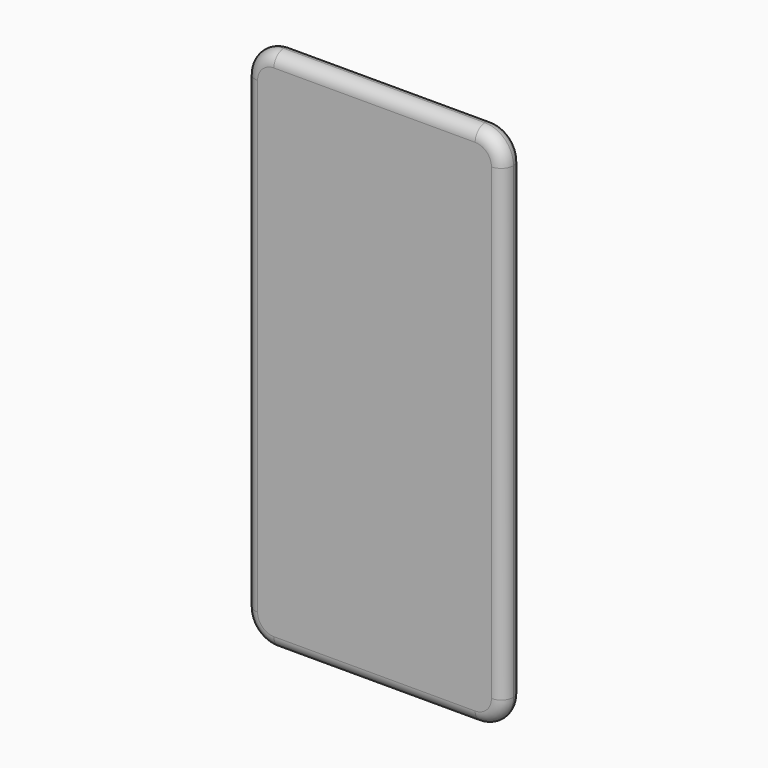
from build123d import *

# Parameters (mm, degrees)
F0_W         = 77.724
F0_H         = 157.988
F1_DEPTH     = 7.112
F2_R         = 8.5849434278
F3_R         = 3.6792614691
F4_T1_DEPTH  = 60.5541131444
F4_T3_DEPTH  = 140.8181131444
F4_T6_ANGLE  = 90
F4_T8_ANGLE  = 90
F4_T10_ANGLE = 90
F4_T12_ANGLE = 90


# Not quite as in the source:
# - a fillet or chamfer that OpenCascade refuses, or shapes differently, is made with other operations: its cross-section is extruded or revolved along the edge and cut away or added


with BuildPart() as f1:
    # F0 (on Front) → F1 (new body)
    with BuildSketch(Plane.XZ):
        with Locations((-9.6872102137, -28.5588150506)):
            Rectangle(F0_W, F0_H)
    extrude(amount=F1_DEPTH)

    # F2
    f2_edges = [f1.edges().sort_by_distance(p)[0] for p in [
        (-48.54921, -3.556, 50.435185),
        (-48.54921, -3.556, -107.552815),
        (29.17479, -3.556, -107.552815),
        (29.17479, -3.556, 50.435185),
    ]]
    fillet(f2_edges, radius=F2_R)

    # F3
    f3_edges = [f1.edges().sort_by_distance(p)[0] for p in [
        (-9.68721, -7.112, 50.435185),
    ]]
    fillet(f3_edges, radius=F3_R)

    # F4: fillet of radius 3.6792614691 on 1 edges, made by hand

    # F4_s2 → F4_t1 (cut)
    with BuildSketch(Plane.YZ.offset(-39.9642667859)):
        with BuildLine():
            ThreePointArc((0, 46.7641917052), (-0.9918847458, 49.2771523705), (-3.4327385309, 50.4351849494))
            Line((-3.4327385309, 50.4351849494), (-3.4278080722, 50.5086048143))
            ThreePointArc((-3.4278080722, 50.5086048143), (-1.7163692655, 50.5087701788), (0, 50.5087701788))
            Line((0, 50.5087701788), (0.0735852294, 50.4351849494))
            Line((0.0735852294, 50.4351849494), (0.0735852294, 46.7641917052))
            Line((0.0735852294, 46.7641917052), (0, 46.7641917052))
        make_face()
        with BuildLine():
            ThreePointArc((-3.4327385309, -107.5528150506), (-0.9918847458, -106.3947824717), (0, -103.8818218065))
            Line((0, -103.8818218065), (0.0735852294, -103.8818218065))
            Line((0.0735852294, -103.8818218065), (0.0735852294, -107.5528150506))
            Line((0.0735852294, -107.5528150506), (0, -107.62640028))
            ThreePointArc((0, -107.62640028), (-1.7163692655, -107.62640028), (-3.4278080722, -107.6262349155))
            Line((-3.4278080722, -107.6262349155), (-3.4327385309, -107.5528150506))
        make_face()
    extrude(amount=F4_T1_DEPTH, mode=Mode.SUBTRACT)

    # F4_s4 → F4_t3 (cut)
    with BuildSketch(Plane.XY.offset(-98.9678716228)):
        with BuildLine():
            ThreePointArc((-44.8782169695, 0), (-47.3911776348, -0.9918847458), (-48.5492102137, -3.4327385309))
            Line((-48.5492102137, -3.4327385309), (-48.6226300785, -3.4278080722))
            ThreePointArc((-48.6226300785, -3.4278080722), (-48.622795443, -1.7163692655), (-48.622795443, 0))
            Line((-48.622795443, 0), (-48.5492102137, 0.0735852294))
            Line((-48.5492102137, 0.0735852294), (-44.8782169695, 0.0735852294))
            Line((-44.8782169695, 0.0735852294), (-44.8782169695, 0))
        make_face()
        with BuildLine():
            ThreePointArc((25.5037965422, 0), (28.0167572074, -0.9918847458), (29.1747897863, -3.4327385309))
            Line((29.1747897863, -3.4327385309), (29.2482096512, -3.4278080722))
            ThreePointArc((29.2482096512, -3.4278080722), (29.2483750157, -1.7163692655), (29.2483750157, 0))
            Line((29.2483750157, 0), (29.1747897863, 0.0735852294))
            Line((29.1747897863, 0.0735852294), (25.5037965422, 0.0735852294))
            Line((25.5037965422, 0.0735852294), (25.5037965422, 0))
        make_face()
    extrude(amount=F4_T3_DEPTH, mode=Mode.SUBTRACT)

    # F4_s5 → F4_t6 (revolve, cut)
    with BuildSketch(Plane.XY.offset(41.8502415216)):
        with BuildLine():
            ThreePointArc((25.5037965422, 0), (28.0167572074, -0.9918847458), (29.1747897863, -3.4327385309))
            Line((29.1747897863, -3.4327385309), (29.2482096512, -3.4278080722))
            ThreePointArc((29.2482096512, -3.4278080722), (29.2483750157, -1.7163692655), (29.2483750157, 0))
            Line((29.2483750157, 0), (29.1747897863, 0.0735852294))
            Line((29.1747897863, 0.0735852294), (25.5037965422, 0.0735852294))
            Line((25.5037965422, 0.0735852294), (25.5037965422, 0))
        make_face()
    revolve(axis=Axis((20.5898463585, 0, 41.8502415216), (0, -1, 0)), revolution_arc=F4_T6_ANGLE, mode=Mode.SUBTRACT)

    # F4_s7 → F4_t8 (revolve, cut)
    with BuildSketch(Plane.YZ.offset(-39.9642667859)):
        with BuildLine():
            ThreePointArc((0, 46.7641917052), (-0.9918847458, 49.2771523705), (-3.4327385309, 50.4351849494))
            Line((-3.4327385309, 50.4351849494), (-3.4278080722, 50.5086048143))
            ThreePointArc((-3.4278080722, 50.5086048143), (-1.7163692655, 50.5087701788), (0, 50.5087701788))
            Line((0, 50.5087701788), (0.0735852294, 50.4351849494))
            Line((0.0735852294, 50.4351849494), (0.0735852294, 46.7641917052))
            Line((0.0735852294, 46.7641917052), (0, 46.7641917052))
        make_face()
    revolve(axis=Axis((-39.9642667859, 0, 41.8502415216), (0, -1, 0)), revolution_arc=F4_T8_ANGLE, mode=Mode.SUBTRACT)

    # F4_s9 → F4_t10 (revolve, cut)
    with BuildSketch(Plane.YZ.offset(-39.9642667859)):
        with BuildLine():
            ThreePointArc((-3.4327385309, -107.5528150506), (-0.9918847458, -106.3947824717), (0, -103.8818218065))
            Line((0, -103.8818218065), (0.0735852294, -103.8818218065))
            Line((0.0735852294, -103.8818218065), (0.0735852294, -107.5528150506))
            Line((0.0735852294, -107.5528150506), (0, -107.62640028))
            ThreePointArc((0, -107.62640028), (-1.7163692655, -107.62640028), (-3.4278080722, -107.6262349155))
            Line((-3.4278080722, -107.6262349155), (-3.4327385309, -107.5528150506))
        make_face()
    revolve(axis=Axis((-39.9642667859, 0, -98.9678716228), (0, 1, 0)), revolution_arc=F4_T10_ANGLE, mode=Mode.SUBTRACT)

    # F4_s11 → F4_t12 (revolve, cut)
    with BuildSketch(Plane.YZ.offset(20.5898463585)):
        with BuildLine():
            ThreePointArc((0, -103.8818218065), (-0.9918847458, -106.3947824717), (-3.4327385309, -107.5528150506))
            Line((-3.4327385309, -107.5528150506), (-3.4278080722, -107.6262349155))
            ThreePointArc((-3.4278080722, -107.6262349155), (-1.7163692655, -107.62640028), (0, -107.62640028))
            Line((0, -107.62640028), (0.0735852294, -107.5528150506))
            Line((0.0735852294, -107.5528150506), (0.0735852294, -103.8818218065))
            Line((0.0735852294, -103.8818218065), (0, -103.8818218065))
        make_face()
    revolve(axis=Axis((20.5898463585, 0, -98.9678716228), (0, -1, 0)), revolution_arc=F4_T12_ANGLE, mode=Mode.SUBTRACT)


solid = f1.part
